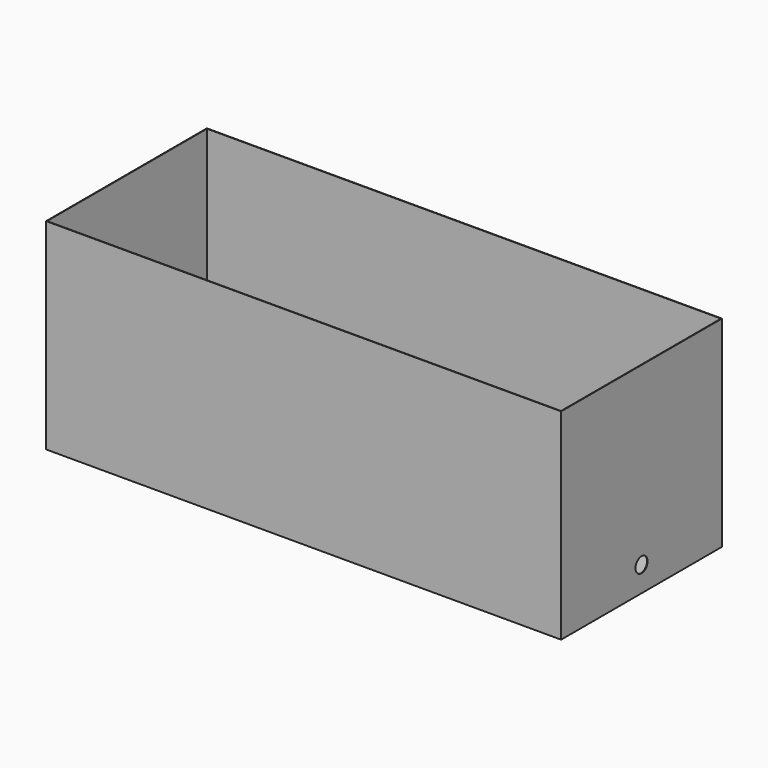
from build123d import *

# Parameters (mm, degrees)
F0_W     = 1025
F0_H     = 400
F1_DEPTH = 400
F2_T     = -1
F5_D     = 40
F8_D     = 30


# Not quite as in the source:
# - the program builds the solid bodies; features that only make, move or delete a surface that nothing else refers to are left out


with BuildPart() as f1:
    # F0 (on Top) → F1 (new body)
    with BuildSketch(Plane.XY):
        Rectangle(F0_W, F0_H)
    extrude(amount=F1_DEPTH)

    # F2
    f2_openings = [f1.faces().sort_by_distance(p)[0] for p in [
        (0, 0, 400),
    ]]
    offset(amount=F2_T, openings=f2_openings)

    # F5 (through all)
    with Locations(Plane.XY.offset(1)):
        with Locations((489.5, 177), (489.5, -177), (-489.5, 177), (-489.5, -177)):
            Hole(F5_D / 2)

    # F8 (through all)
    with Locations(Plane(origin=(-512.5, 0, 0), x_dir=(0, -1, 0), z_dir=(-1, 0, 0))):
        with Locations((0, 50)):
            Hole(F8_D / 2)


solid = f1.part
